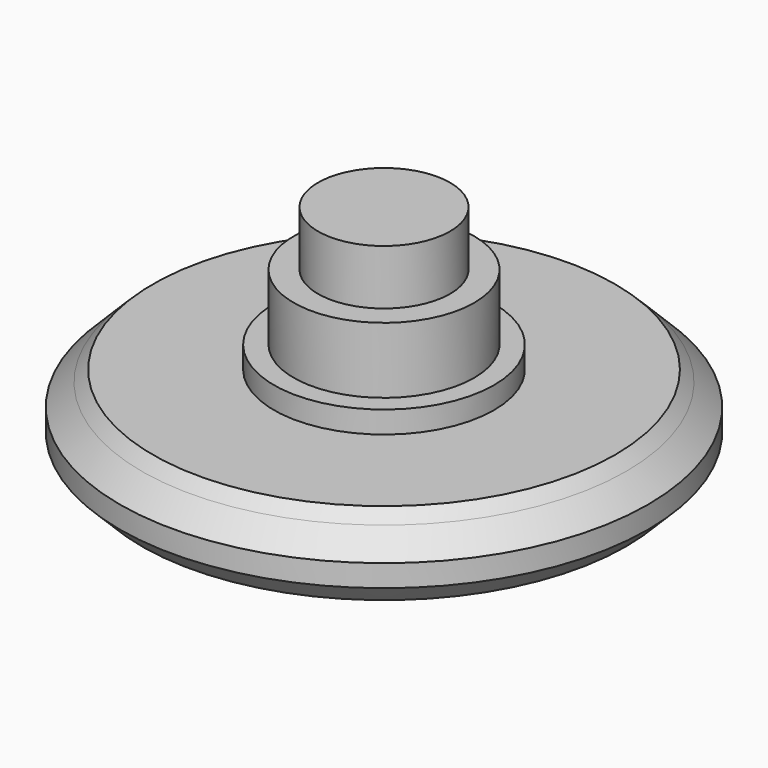
from build123d import *

# Parameters (mm, degrees)
F0_R     = 12
F0_R_2   = 11
F0_R_3   = 5
F0_R_4   = 4.1
F0_R_5   = 3
F1_DEPTH = 2
F2_DEPTH = 3.5
F3_SIZE  = 0.99999
F4_DEPTH = 4.5
F5_DEPTH = 7.5
F6_DEPTH = 10
F7_SIZE  = 1
F8_SIZE  = 0.5


# Not quite as in the source:
# - a fillet or chamfer is up to 0.001 mm smaller than in the source, because OpenCascade refuses the exact size


with BuildPart() as f1:
    # F0 (on Top) → F1 (new body)
    with BuildSketch(Plane.XY):
        Circle(F0_R)
        Circle(F0_R_2, mode=Mode.SUBTRACT)
        Circle(F0_R_2)
        Circle(F0_R_3, mode=Mode.SUBTRACT)
        Circle(F0_R_3)
        Circle(F0_R_4, mode=Mode.SUBTRACT)
        Circle(F0_R_4)
        Circle(F0_R_5, mode=Mode.SUBTRACT)
        Circle(F0_R_5)
    extrude(amount=F1_DEPTH)

    # F0 (on Top) → F2 (join)
    with BuildSketch(Plane.XY):
        Circle(F0_R_2)
        Circle(F0_R_3, mode=Mode.SUBTRACT)
        Circle(F0_R_3)
        Circle(F0_R_4, mode=Mode.SUBTRACT)
        Circle(F0_R_4)
        Circle(F0_R_5, mode=Mode.SUBTRACT)
        Circle(F0_R_5)
    extrude(amount=F2_DEPTH)

    # F3 (size 1 in the source; OpenCascade refuses exactly that, so slightly less here)
    f3_edges = [f1.edges().sort_by_distance(p)[0] for p in [
        (-11, 0, 2),
    ]]
    chamfer(f3_edges, length=F3_SIZE)

    # F0 (on Top) → F4 (join)
    with BuildSketch(Plane.XY):
        Circle(F0_R_3)
        Circle(F0_R_4, mode=Mode.SUBTRACT)
        Circle(F0_R_4)
        Circle(F0_R_5, mode=Mode.SUBTRACT)
        Circle(F0_R_5)
    extrude(amount=F4_DEPTH)

    # F0 (on Top) → F5 (join)
    with BuildSketch(Plane.XY):
        Circle(F0_R_4)
        Circle(F0_R_5, mode=Mode.SUBTRACT)
    extrude(amount=F5_DEPTH)

    # F0 (on Top) → F6 (join)
    with BuildSketch(Plane.XY):
        Circle(F0_R_5)
    extrude(amount=F6_DEPTH)

    # F7
    f7_edges = [f1.edges().sort_by_distance(p)[0] for p in [
        (-12, 0, 0),
    ]]
    chamfer(f7_edges, length=F7_SIZE)

    # F8
    f8_edges = [f1.edges().sort_by_distance(p)[0] for p in [
        (-11, 0, 3.5),
    ]]
    chamfer(f8_edges, length=F8_SIZE)


solid = f1.part
